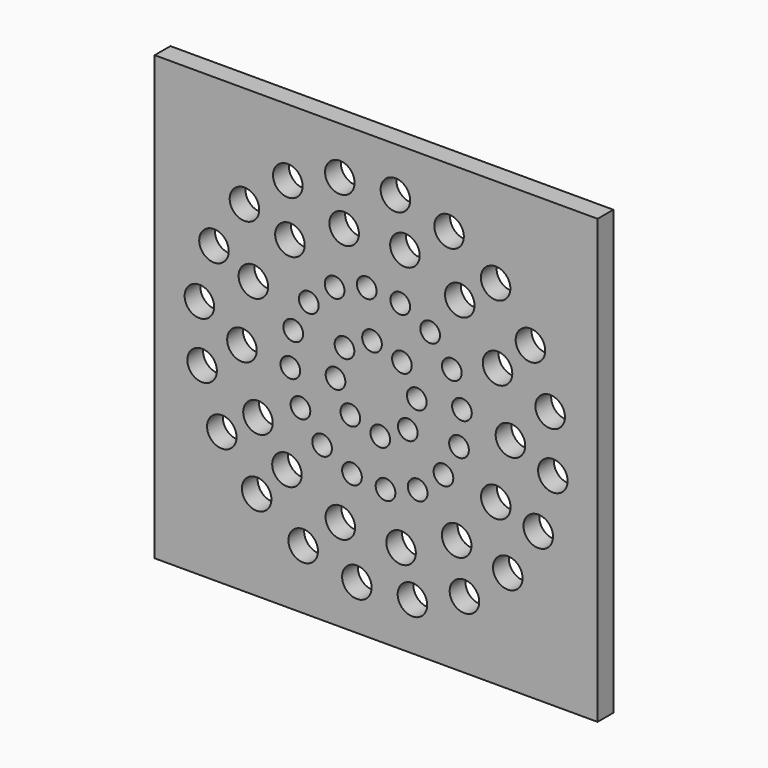
from build123d import *

# Parameters (mm, degrees)
F0_W     = 45
F0_H     = 45
F1_DEPTH = 2
F2_R     = 1
F2_R_2   = 1.5
F3_DEPTH = 19.6
F4_DEPTH = 25


# Not quite as in the source:
# - a feature names something its author has since deleted; it is built from what else it names


with BuildPart() as f1:
    # F0 (on Front) → F1 (new body)
    with BuildSketch(Plane.XZ):
        with Locations((-22.5, 22.5)):
            Rectangle(F0_W, F0_H)
    extrude(amount=F1_DEPTH)

    # F2 (on face) → F3 (cut)
    with BuildSketch(Plane.XZ.offset(2)):
        with Locations((-26.6271115437, 22.0804515862)):
            Circle(F2_R)
        with Locations((-25.7149740877, 25.1216430309)):
            Circle(F2_R)
        with Locations((-22.9195484138, 26.6271115437)):
            Circle(F2_R)
        with Locations((-25.1216430309, 19.2850259123)):
            Circle(F2_R)
        with Locations((-10.3415464992, 16.307327403)):
            Circle(F2_R_2)
        with Locations((-8.8567808269, 22.3006108876)):
            Circle(F2_R_2)
        with Locations((-10.1657718628, 28.3347237882)):
            Circle(F2_R_2)
        with Locations((-14.0004741816, 33.1740454509)):
            Circle(F2_R_2)
        with Locations((-34.5032584426, 16.011627925)):
            Circle(F2_R_2)
        with Locations((-40.4566549108, 24.4574602037)):
            Circle(F2_R_2)
        with Locations((-40.1826821325, 18.8127437526)):
            Circle(F2_R_2)
        with Locations((-29.9105668117, 6.027094805)):
            Circle(F2_R_2)
        with Locations((-19.5756460311, 35.8276156641)):
            Circle(F2_R_2)
        with Locations((-18.8127437526, 4.8173178675)):
            Circle(F2_R_2)
        with Locations((-38.1778052247, 13.5289616335)):
            Circle(F2_R_2)
        with Locations((-34.6382755077, 9.1233272547)):
            Circle(F2_R_2)
        with Locations((-24.4574602037, 4.5433450892)):
            Circle(F2_R_2)
        with Locations((-25.7496452846, 35.7520561027)):
            Circle(F2_R_2)
        with Locations((-31.2582064036, 32.9628392904)):
            Circle(F2_R_2)
        with Locations((-38.972905195, 29.9105668117)):
            Circle(F2_R_2)
        with Locations((-36.1342532423, 21.9667796436)):
            Circle(F2_R_2)
        with Locations((-34.9733273102, 28.0311202515)):
            Circle(F2_R_2)
        with Locations((-13.5289616335, 6.8221947753)):
            Circle(F2_R_2)
        with Locations((-26.1872562474, 40.1826821325)):
            Circle(F2_R_2)
        with Locations((-31.4710383665, 38.1778052247)):
            Circle(F2_R_2)
        with Locations((-35.8766727453, 34.6382755077)):
            Circle(F2_R_2)
        with Locations((-9.1233272547, 10.3617244923)):
            Circle(F2_R_2)
        with Locations((-6.027094805, 15.0894331883)):
            Circle(F2_R_2)
        with Locations((-4.5433450892, 20.5425397963)):
            Circle(F2_R_2)
        with Locations((-4.8173178675, 26.1872562474)):
            Circle(F2_R_2)
    extrude(amount=-F3_DEPTH, mode=Mode.SUBTRACT)

    # F2 (on face) → F4 (cut)
    with BuildSketch(Plane.XZ.offset(2)):
        with Locations((-22.9195484138, 26.6271115437)):
            Circle(F2_R)
        with Locations((-25.7149740877, 25.1216430309)):
            Circle(F2_R)
        with Locations((-26.6271115437, 22.0804515862)):
            Circle(F2_R)
        with Locations((-25.1216430309, 19.2850259123)):
            Circle(F2_R)
        with Locations((-34.5032584426, 16.011627925)):
            Circle(F2_R_2)
        with Locations((-36.1342532423, 21.9667796436)):
            Circle(F2_R_2)
        with Locations((-34.9733273102, 28.0311202515)):
            Circle(F2_R_2)
        with Locations((-31.2582064036, 32.9628392904)):
            Circle(F2_R_2)
        with Locations((-25.7496452846, 35.7520561027)):
            Circle(F2_R_2)
        with Locations((-19.5756460311, 35.8276156641)):
            Circle(F2_R_2)
        with Locations((-14.0004741816, 33.1740454509)):
            Circle(F2_R_2)
        with Locations((-10.1657718628, 28.3347237882)):
            Circle(F2_R_2)
        with Locations((-8.8567808269, 22.3006108876)):
            Circle(F2_R_2)
        with Locations((-10.3415464992, 16.307327403)):
            Circle(F2_R_2)
        with Locations((-26.1872562474, 40.1826821325)):
            Circle(F2_R_2)
        with Locations((-31.4710383665, 38.1778052247)):
            Circle(F2_R_2)
        with Locations((-35.8766727453, 34.6382755077)):
            Circle(F2_R_2)
        with Locations((-38.972905195, 29.9105668117)):
            Circle(F2_R_2)
        with Locations((-40.4566549108, 24.4574602037)):
            Circle(F2_R_2)
        with Locations((-40.1826821325, 18.8127437526)):
            Circle(F2_R_2)
        with Locations((-38.1778052247, 13.5289616335)):
            Circle(F2_R_2)
        with Locations((-34.6382755077, 9.1233272547)):
            Circle(F2_R_2)
        with Locations((-29.9105668117, 6.027094805)):
            Circle(F2_R_2)
        with Locations((-24.4574602037, 4.5433450892)):
            Circle(F2_R_2)
        with Locations((-18.8127437526, 4.8173178675)):
            Circle(F2_R_2)
        with Locations((-13.5289616335, 6.8221947753)):
            Circle(F2_R_2)
        with Locations((-9.1233272547, 10.3617244923)):
            Circle(F2_R_2)
        with Locations((-6.027094805, 15.0894331883)):
            Circle(F2_R_2)
        with Locations((-4.5433450892, 20.5425397963)):
            Circle(F2_R_2)
        with Locations((-4.8173178675, 26.1872562474)):
            Circle(F2_R_2)
        with Locations((-14.3160296348, 11.5821332447)):
            Circle(F2_R_2)
        with Locations((-19.966365208, 9.0926184449)):
            Circle(F2_R_2)
        with Locations((-26.1355196249, 9.3485672841)):
            Circle(F2_R_2)
        with Locations((-31.5602194369, 12.2975684673)):
            Circle(F2_R_2)
        with Locations((-6.8221947753, 31.4710383665)):
            Circle(F2_R_2)
        with Locations((-10.3617244923, 35.8766727453)):
            Circle(F2_R_2)
        with Locations((-15.0894331883, 38.972905195)):
            Circle(F2_R_2)
        with Locations((-20.5425397963, 40.4566549108)):
            Circle(F2_R_2)
        with Locations((-26.7185367273, 30.1892252677)):
            Circle(F2_R)
        with Locations((-29.3399588572, 27.9895537314)):
            Circle(F2_R)
        with Locations((-30.9200592554, 24.9541474023)):
            Circle(F2_R)
        with Locations((-31.2182819601, 21.5451193782)):
            Circle(F2_R)
        with Locations((-30.1892252677, 18.2814632727)):
            Circle(F2_R)
        with Locations((-27.9895537314, 15.6600411428)):
            Circle(F2_R)
        with Locations((-24.9541474023, 14.0799407446)):
            Circle(F2_R)
        with Locations((-21.5451193782, 13.7817180399)):
            Circle(F2_R)
        with Locations((-18.2814632727, 14.8107747323)):
            Circle(F2_R)
        with Locations((-15.6600411428, 17.0104462686)):
            Circle(F2_R)
        with Locations((-22.0804515862, 18.3728884563)):
            Circle(F2_R)
        with Locations((-19.2850259123, 19.8783569691)):
            Circle(F2_R)
        with Locations((-18.3728884563, 22.9195484138)):
            Circle(F2_R)
        with Locations((-19.8783569691, 25.7149740877)):
            Circle(F2_R)
        with Locations((-14.0799407446, 20.0458525977)):
            Circle(F2_R)
        with Locations((-13.7817180399, 23.4548806218)):
            Circle(F2_R)
        with Locations((-14.8107747323, 26.7185367273)):
            Circle(F2_R)
        with Locations((-17.0104462686, 29.3399588572)):
            Circle(F2_R)
        with Locations((-20.0458525977, 30.9200592554)):
            Circle(F2_R)
        with Locations((-23.4548806218, 31.2182819601)):
            Circle(F2_R)
    extrude(amount=-F4_DEPTH, mode=Mode.SUBTRACT)


solid = f1.part
